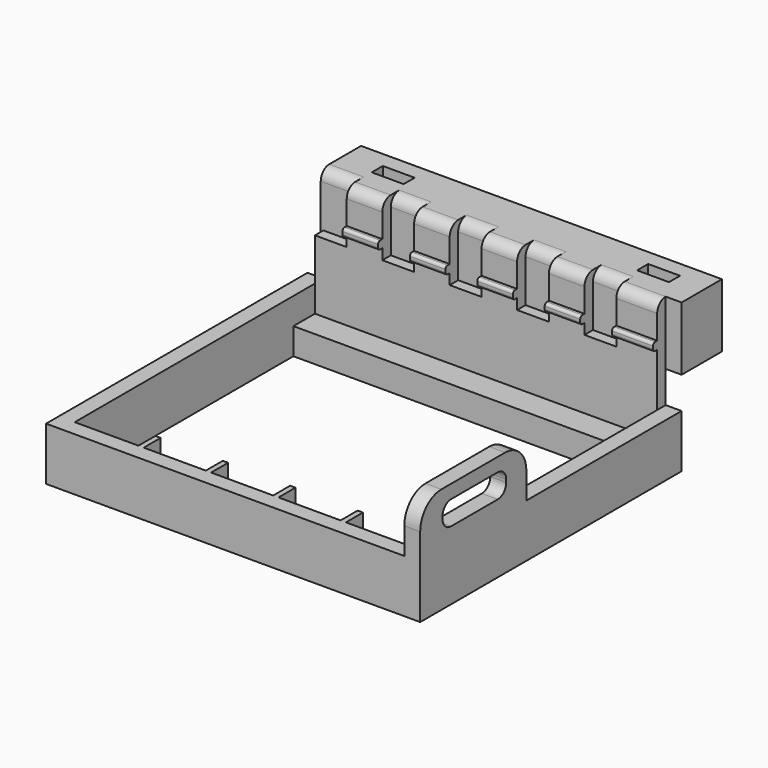
from build123d import *

# Parameters (mm, degrees)
F0_W      = 70.5
F0_H      = 61.57
F0_W_2    = 1
F0_H_2    = 4
F1_DEPTH  = 10
F0_W_3    = 64.5
F0_H_3    = 5.07
F2_DEPTH  = 5
F3_W      = 64.5
F3_H      = 2
F4_DEPTH  = 18
F5_W      = 1
F5_H      = 1.5
F6_DEPTH  = 64.5
F7_R      = 0.5
F8_W      = 6
F8_H      = 9.142870052
F9_DEPTH  = 10
F10_W     = 9.5
F10_H     = 12
F11_DEPTH = 68
F13_DEPTH = 4
F14_W     = 6
F14_H     = 2.6
F15_DEPTH = 11
F17_DEPTH = 10
F18_W     = 15
F18_H     = 4.5
F19_DEPTH = 25
F20_R     = 5
F21_R     = 1.99999


# Not quite as in the source:
# - a fillet or chamfer is up to 0.001 mm smaller than in the source, because OpenCascade refuses the exact size


with BuildPart() as f1:
    # F0 (on Top) → F1 (new body)
    with BuildSketch(Plane.XY):
        with Locations((20.3630310733, 4.7424566842)):
            Rectangle(F0_W, F0_H)
        Polygon((-11.8869689267, 28.4574566842), (-11.8869689267, 33.5274566842), (52.6130310733, 33.5274566842), (52.6130310733, 28.4574566842), (52.6130310733, -23.0425433158), (39.2130310733, -23.0425433158), (38.2130310733, -23.0425433158), (26.5130310733, -23.0425433158), (25.5130310733, -23.0425433158), (13.8130310733, -23.0425433158), (12.8130310733, -23.0425433158), (1.1130310733, -23.0425433158), (0.1130310733, -23.0425433158), (-11.8869689267, -23.0425433158), align=None, mode=Mode.SUBTRACT)
        with Locations((0.6130310733, -21.0425433158)):
            Rectangle(F0_W_2, F0_H_2)
        with Locations((13.3130310733, -21.0425433158)):
            Rectangle(F0_W_2, F0_H_2)
        with Locations((26.0130310733, -21.0425433158)):
            Rectangle(F0_W_2, F0_H_2)
        with Locations((38.7130310733, -21.0425433158)):
            Rectangle(F0_W_2, F0_H_2)
    extrude(amount=F1_DEPTH)

    # F0 (on Top) → F2 (join)
    with BuildSketch(Plane.XY):
        with Locations((20.3630310733, 30.9924566842)):
            Rectangle(F0_W_3, F0_H_3)
    extrude(amount=F2_DEPTH)

    # F3 (on face) → F4 (join)
    with BuildSketch(Plane.XY.offset(10)):
        with Locations((20.3630310733, 34.5274566842)):
            Rectangle(F3_W, F3_H)
    extrude(amount=F4_DEPTH)

    # F5 (on face) → F6 (join)
    with BuildSketch(Plane.YZ.offset(52.6130310733)):
        with Locations((33.0274566842, 20.75)):
            Rectangle(F5_W, F5_H)
    extrude(amount=-F6_DEPTH)

    # F7
    f7_edges = [f1.edges().sort_by_distance(p)[0] for p in [
        (20.363031, 32.527457, 21.5),
        (20.363031, 32.527457, 20),
    ]]
    fillet(f7_edges, radius=F7_R)

    # F8 (on face) → F9 (cut)
    with BuildSketch(Plane.XY.offset(28)):
        with Locations((-8.8869689267, 30.9560216582)):
            Rectangle(F8_W, F8_H)
        with Locations((3.8130310733, 30.9560216582)):
            Rectangle(F8_W, F8_H)
        with Locations((16.5130310733, 30.9560216582)):
            Rectangle(F8_W, F8_H)
        with Locations((29.2130310733, 30.9560216582)):
            Rectangle(F8_W, F8_H)
        with Locations((41.9130310733, 30.9560216582)):
            Rectangle(F8_W, F8_H)
    extrude(amount=-F9_DEPTH, mode=Mode.SUBTRACT)

    # F10 (on face) → F11 (join)
    with BuildSketch(Plane.YZ.offset(55.6130310733)):
        with Locations((40.2774566842, 22)):
            Rectangle(F10_W, F10_H)
    extrude(amount=-F11_DEPTH)

    # F12 (on face) → F13 (cut)
    with BuildSketch(Plane(origin=(0, 45.0274566842, 0), x_dir=(-1, 0, 0), z_dir=(0, 1, 0))):
        with BuildLine():
            ThreePointArc((-48.4359067289, 21.5), (-48.9359067289, 20.8228756555), (-49.1130310733, 20))
            ThreePointArc((-49.1130310733, 20), (-47.1130310733, 18), (-45.1130310733, 20))
            ThreePointArc((-45.1130310733, 20), (-45.2901554178, 20.8228756555), (-45.7901554178, 21.5))
            ThreePointArc((-45.7901554178, 21.5), (-47.1130310733, 21), (-48.4359067289, 21.5))
        make_face()
        with BuildLine():
            Line((-49.1130310733, 23), (-49.1130310733, 20))
            ThreePointArc((-49.1130310733, 20), (-48.9359067289, 20.8228756555), (-48.4359067289, 21.5))
            ThreePointArc((-48.4359067289, 21.5), (-48.9359067289, 22.1771243445), (-49.1130310733, 23))
        make_face()
        with BuildLine():
            ThreePointArc((-45.7901554178, 21.5), (-45.2901554178, 20.8228756555), (-45.1130310733, 20))
            Line((-45.1130310733, 20), (-45.1130310733, 23))
            ThreePointArc((-45.1130310733, 23), (-45.2901554178, 22.1771243445), (-45.7901554178, 21.5))
        make_face()
        with BuildLine():
            ThreePointArc((-49.1130310733, 23), (-48.9359067289, 22.1771243445), (-48.4359067289, 21.5))
            ThreePointArc((-48.4359067289, 21.5), (-47.1130310733, 22), (-45.7901554178, 21.5))
            ThreePointArc((-45.7901554178, 21.5), (-45.2901554178, 22.1771243445), (-45.1130310733, 23))
            ThreePointArc((-45.1130310733, 23), (-47.1130310733, 25), (-49.1130310733, 23))
        make_face()
        with BuildLine():
            ThreePointArc((1.5640932711, 21.5), (1.0640932711, 20.8228756555), (0.8869689267, 20))
            ThreePointArc((0.8869689267, 20), (2.8869689267, 18), (4.8869689267, 20))
            ThreePointArc((4.8869689267, 20), (4.7098445822, 20.8228756555), (4.2098445822, 21.5))
            ThreePointArc((4.2098445822, 21.5), (2.8869689267, 21), (1.5640932711, 21.5))
        make_face()
        with BuildLine():
            Line((0.8869689267, 23), (0.8869689267, 20))
            ThreePointArc((0.8869689267, 20), (1.0640932711, 20.8228756555), (1.5640932711, 21.5))
            ThreePointArc((1.5640932711, 21.5), (1.0640932711, 22.1771243445), (0.8869689267, 23))
        make_face()
        with BuildLine():
            ThreePointArc((4.2098445822, 21.5), (4.7098445822, 20.8228756555), (4.8869689267, 20))
            Line((4.8869689267, 20), (4.8869689267, 23))
            ThreePointArc((4.8869689267, 23), (4.7098445822, 22.1771243445), (4.2098445822, 21.5))
        make_face()
        with BuildLine():
            ThreePointArc((0.8869689267, 23), (1.0640932711, 22.1771243445), (1.5640932711, 21.5))
            ThreePointArc((1.5640932711, 21.5), (2.8869689267, 22), (4.2098445822, 21.5))
            ThreePointArc((4.2098445822, 21.5), (4.7098445822, 22.1771243445), (4.8869689267, 23))
            ThreePointArc((4.8869689267, 23), (2.8869689267, 25), (0.8869689267, 23))
        make_face()
        with BuildLine():
            ThreePointArc((-45.7901554178, 21.5), (-47.1130310733, 22), (-48.4359067289, 21.5))
            ThreePointArc((-48.4359067289, 21.5), (-47.1130310733, 21), (-45.7901554178, 21.5))
        make_face()
        with BuildLine():
            ThreePointArc((4.2098445822, 21.5), (2.8869689267, 22), (1.5640932711, 21.5))
            ThreePointArc((1.5640932711, 21.5), (2.8869689267, 21), (4.2098445822, 21.5))
        make_face()
    extrude(amount=-F13_DEPTH, mode=Mode.SUBTRACT)

    # F14 (on face) → F15 (cut)
    with BuildSketch(Plane.XY.offset(28)):
        with Locations((-2.8869689267, 40.7274566842)):
            Rectangle(F14_W, F14_H)
        with Locations((47.1130310733, 40.7274566842)):
            Rectangle(F14_W, F14_H)
    extrude(amount=-F15_DEPTH, mode=Mode.SUBTRACT)

    # F16 (on face) → F17 (join)
    with BuildSketch(Plane.XY.offset(10)):
        Polygon((52.6130310733, -26.0425433158), (55.6130310733, -26.0425433158), (55.6130310733, -1.0425433158), (52.6130310733, -1.0425433158), (52.6130310733, -23.0425433158), align=None)
    extrude(amount=F17_DEPTH)

    # F18 (on face) → F19 (cut)
    with BuildSketch(Plane.YZ.offset(55.6130310733)):
        with Locations((-13.2769846171, 15.1880288571)):
            Rectangle(F18_W, F18_H)
    extrude(amount=-F19_DEPTH, mode=Mode.SUBTRACT)

    # F20
    f20_edges = [f1.edges().sort_by_distance(p)[0] for p in [
        (54.113031, -1.042543, 20),
        (54.113031, -26.042543, 20),
    ]]
    fillet(f20_edges, radius=F20_R)

    # F21 (radius 2 in the source; OpenCascade refuses exactly that, so slightly less here)
    f21_edges = [f1.edges().sort_by_distance(p)[0] for p in [
        (54.113031, -20.776985, 17.438029),
        (54.113031, -20.776985, 12.938029),
        (54.113031, -5.776985, 12.938029),
        (54.113031, -5.776985, 17.438029),
        (41.913031, 35.527457, 28),
        (48.763031, 33.527457, 28),
        (35.563031, 33.527457, 28),
        (29.213031, 35.527457, 28),
        (22.863031, 33.527457, 28),
        (16.513031, 35.527457, 28),
        (10.163031, 33.527457, 28),
        (3.813031, 35.527457, 28),
        (-2.536969, 33.527457, 28),
        (-9.136969, 35.527457, 28),
    ]]
    fillet(f21_edges, radius=F21_R)


solid = f1.part
